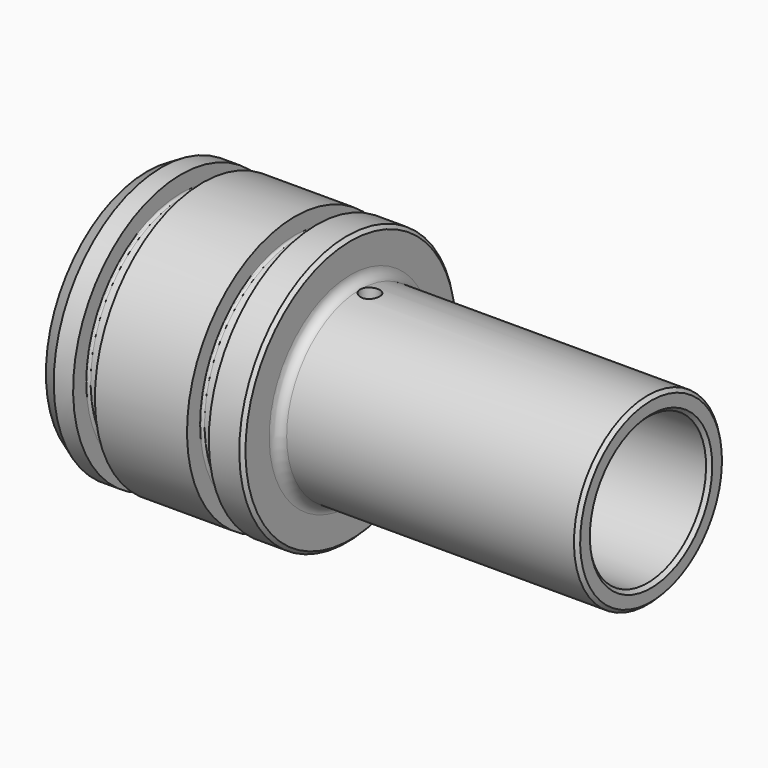
from build123d import *

# Parameters (mm, degrees)
F2_R     = 3.175
F4_R     = 0.79375
F5_R     = 3.175
F6_DEPTH = 50.8


# Not quite as in the source:
# - a fillet or chamfer that OpenCascade refuses, or shapes differently, is made with other operations: its cross-section is extruded or revolved along the edge and cut away or added


with BuildPart() as f1:
    # F0 (on Front) → F1 (revolve)
    with BuildSketch(Plane.XZ):
        Polygon((0, 25.0620320151), (1.1225320151, 23.9395), (15.875, 23.9395), (15.875, 27.6225), (19.05, 27.6225), (19.05, 23.9395), (28.575, 23.9395), (28.575, 27.6225), (31.75, 27.6225), (31.75, 23.9395), (47.625, 23.9395), (47.625, 25.4), (82.55, 25.4), (82.55, 23.9395), (163.9774679849, 23.9395), (165.1, 25.0620320151), (165.1, 29.0399679849), (163.9774679849, 30.1625), (66.675, 30.1625), (66.675, 43.0734679849), (65.5524679849, 44.196), (55.5625, 44.196), (55.5625, 38.0238), (48.4251, 38.0238), (48.4251, 44.196), (18.2499, 44.196), (18.2499, 38.0238), (11.1125, 38.0238), (11.1125, 44.196), (4.7625, 44.196), (0, 41.446369343), align=None)
    revolve(axis=Axis((55.6648539445, 0, 0), (1, 0, 0)))

    # F2
    f2_edges = [f1.edges().sort_by_distance(p)[0] for p in [
        (66.675, 0, -30.1625),
    ]]
    fillet(f2_edges, radius=F2_R)

    # F3: fillet of radius 1.5875 on 2 edges, made by hand

    # F3_s1 → F3_t2 (revolve)
    with BuildSketch(Plane.XZ):
        with BuildLine():
            ThreePointArc((49.2074118459, 25.4), (48.1307169611, 24.97906949), (47.625, 23.9395))
            Line((47.625, 23.9395), (47.625, 25.4))
            Line((47.625, 25.4), (49.2074118459, 25.4))
        make_face()
    revolve(axis=Axis((47.625, 0, 0), (1, 0, 0)))

    # F3_s3 → F3_t4 (revolve)
    with BuildSketch(Plane.XZ):
        with BuildLine():
            ThreePointArc((82.55, 23.9395), (82.0442830389, 24.97906949), (80.9675881541, 25.4))
            Line((80.9675881541, 25.4), (82.55, 25.4))
            Line((82.55, 25.4), (82.55, 23.9395))
        make_face()
    revolve(axis=Axis((82.55, 0, 0), (1, 0, 0)))

    # F4
    f4_edges = [f1.edges().sort_by_distance(p)[0] for p in [
        (18.2499, 0, -38.0238),
        (55.5625, 0, -38.0238),
        (19.05, 0, -27.6225),
        (31.75, 0, -27.6225),
        (15.875, 0, -27.6225),
        (28.575, 0, -27.6225),
        (11.1125, 0, -38.0238),
        (48.4251, 0, -38.0238),
    ]]
    fillet(f4_edges, radius=F4_R)

    # F5 (on Top) → F6 (cut, symmetric)
    with BuildSketch(Plane.XY):
        with Locations((73.025, 0)):
            Circle(F5_R)
    extrude(amount=F6_DEPTH, both=True, mode=Mode.SUBTRACT)


solid = f1.part
